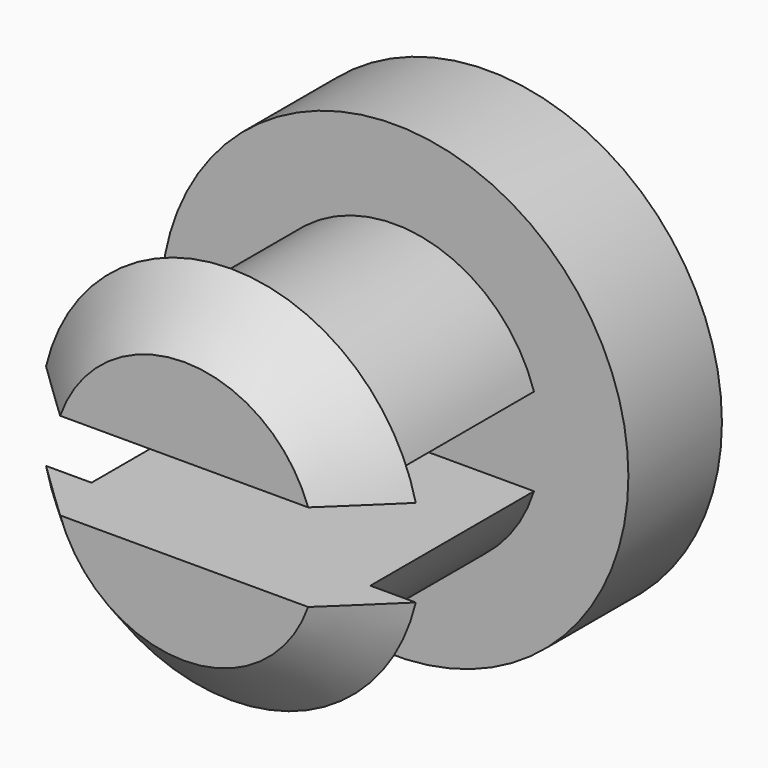
from build123d import *

# Parameters (mm, degrees)
F0_R     = 4
F1_DEPTH = 2
F2_DEPTH = 5.5
F3_START = 5.5
F3_DEPTH = 1
F4_SIZE  = 0.99999


# Not quite as in the source:
# - a fillet or chamfer is up to 0.001 mm smaller than in the source, because OpenCascade refuses the exact size


with BuildPart() as f1:
    # F0 (on Front) → F1 (new body)
    with BuildSketch(Plane.XZ):
        Circle(F0_R)
        with BuildLine():
            ThreePointArc((-3.1622776602, 0.75), (0, 3.25), (3.1622776602, 0.75))
            Line((3.1622776602, 0.75), (3.5, 0.75))
            Line((3.5, 0.75), (3.5, -0.75))
            Line((3.5, -0.75), (3.1622776602, -0.75))
            ThreePointArc((3.1622776602, -0.75), (0, -3.25), (-3.1622776602, -0.75))
            Line((-3.1622776602, -0.75), (-3.5, -0.75))
            Line((-3.5, -0.75), (-3.5, 0.75))
            Line((-3.5, 0.75), (-3.1622776602, 0.75))
        make_face(mode=Mode.SUBTRACT)
        with BuildLine():
            ThreePointArc((2.3848480035, -0.75), (2.4710443145, -0.3793942482), (2.5, 0))
            ThreePointArc((2.5, 0), (2.4710443145, 0.3793942482), (2.3848480035, 0.75))
            Line((2.3848480035, 0.75), (-2.3848480035, 0.75))
            ThreePointArc((-2.3848480035, 0.75), (-2.5, 0), (-2.3848480035, -0.75))
            Line((-2.3848480035, -0.75), (2.3848480035, -0.75))
        make_face()
        with BuildLine():
            ThreePointArc((-2.3848480035, -0.75), (0, -2.5), (2.3848480035, -0.75))
            Line((2.3848480035, -0.75), (-2.3848480035, -0.75))
        make_face()
        with BuildLine():
            Line((-2.3848480035, 0.75), (2.3848480035, 0.75))
            ThreePointArc((2.3848480035, 0.75), (0, 2.5), (-2.3848480035, 0.75))
        make_face()
        with BuildLine():
            Line((3.1622776602, -0.75), (2.3848480035, -0.75))
            ThreePointArc((2.3848480035, -0.75), (0, -2.5), (-2.3848480035, -0.75))
            Line((-2.3848480035, -0.75), (-3.1622776602, -0.75))
            ThreePointArc((-3.1622776602, -0.75), (0, -3.25), (3.1622776602, -0.75))
        make_face()
        with BuildLine():
            ThreePointArc((-2.3848480035, 0.75), (0, 2.5), (2.3848480035, 0.75))
            Line((2.3848480035, 0.75), (3.1622776602, 0.75))
            ThreePointArc((3.1622776602, 0.75), (0, 3.25), (-3.1622776602, 0.75))
            Line((-3.1622776602, 0.75), (-2.3848480035, 0.75))
        make_face()
        with BuildLine():
            ThreePointArc((-2.3848480035, -0.75), (-2.5, 0), (-2.3848480035, 0.75))
            Line((-2.3848480035, 0.75), (-3.1622776602, 0.75))
            ThreePointArc((-3.1622776602, 0.75), (-3.25, 0), (-3.1622776602, -0.75))
            Line((-3.1622776602, -0.75), (-2.3848480035, -0.75))
        make_face()
        with BuildLine():
            ThreePointArc((2.3848480035, 0.75), (2.4710443145, 0.3793942482), (2.5, 0))
            ThreePointArc((2.5, 0), (2.4710443145, -0.3793942482), (2.3848480035, -0.75))
            Line((2.3848480035, -0.75), (3.1622776602, -0.75))
            ThreePointArc((3.1622776602, -0.75), (3.2279949191, -0.3775563564), (3.25, 0))
            ThreePointArc((3.25, 0), (3.2279949191, 0.3775563564), (3.1622776602, 0.75))
            Line((3.1622776602, 0.75), (2.3848480035, 0.75))
        make_face()
        with BuildLine():
            Line((3.5, 0.75), (3.1622776602, 0.75))
            ThreePointArc((3.1622776602, 0.75), (3.2279949191, 0.3775563564), (3.25, 0))
            ThreePointArc((3.25, 0), (3.2279949191, -0.3775563564), (3.1622776602, -0.75))
            Line((3.1622776602, -0.75), (3.5, -0.75))
            Line((3.5, -0.75), (3.5, 0.75))
        make_face()
        with BuildLine():
            ThreePointArc((-3.1622776602, -0.75), (-3.25, 0), (-3.1622776602, 0.75))
            Line((-3.1622776602, 0.75), (-3.5, 0.75))
            Line((-3.5, 0.75), (-3.5, -0.75))
            Line((-3.5, -0.75), (-3.1622776602, -0.75))
        make_face()
    extrude(amount=F1_DEPTH)

    # F0 (on Front) → F2 (join)
    with BuildSketch(Plane.XZ):
        with BuildLine():
            Line((-2.3848480035, 0.75), (2.3848480035, 0.75))
            ThreePointArc((2.3848480035, 0.75), (0, 2.5), (-2.3848480035, 0.75))
        make_face()
        with BuildLine():
            ThreePointArc((-2.3848480035, -0.75), (0, -2.5), (2.3848480035, -0.75))
            Line((2.3848480035, -0.75), (-2.3848480035, -0.75))
        make_face()
    extrude(amount=F2_DEPTH)

    # F0 (on Front) → F3 (join)
    with BuildSketch(Plane.XZ.offset(F3_START)):
        with BuildLine():
            Line((3.1622776602, -0.75), (2.3848480035, -0.75))
            ThreePointArc((2.3848480035, -0.75), (0, -2.5), (-2.3848480035, -0.75))
            Line((-2.3848480035, -0.75), (-3.1622776602, -0.75))
            ThreePointArc((-3.1622776602, -0.75), (0, -3.25), (3.1622776602, -0.75))
        make_face()
        with BuildLine():
            ThreePointArc((-2.3848480035, 0.75), (0, 2.5), (2.3848480035, 0.75))
            Line((2.3848480035, 0.75), (3.1622776602, 0.75))
            ThreePointArc((3.1622776602, 0.75), (0, 3.25), (-3.1622776602, 0.75))
            Line((-3.1622776602, 0.75), (-2.3848480035, 0.75))
        make_face()
        with BuildLine():
            Line((-2.3848480035, 0.75), (2.3848480035, 0.75))
            ThreePointArc((2.3848480035, 0.75), (0, 2.5), (-2.3848480035, 0.75))
        make_face()
        with BuildLine():
            ThreePointArc((-2.3848480035, -0.75), (0, -2.5), (2.3848480035, -0.75))
            Line((2.3848480035, -0.75), (-2.3848480035, -0.75))
        make_face()
    extrude(amount=F3_DEPTH)

    # F4 (size 1 in the source; OpenCascade refuses exactly that, so slightly less here)
    f4_edges = [f1.edges().sort_by_distance(p)[0] for p in [
        (0, -6.5, 3.25),
        (0, -6.5, -3.25),
    ]]
    chamfer(f4_edges, length=F4_SIZE)


solid = f1.part
